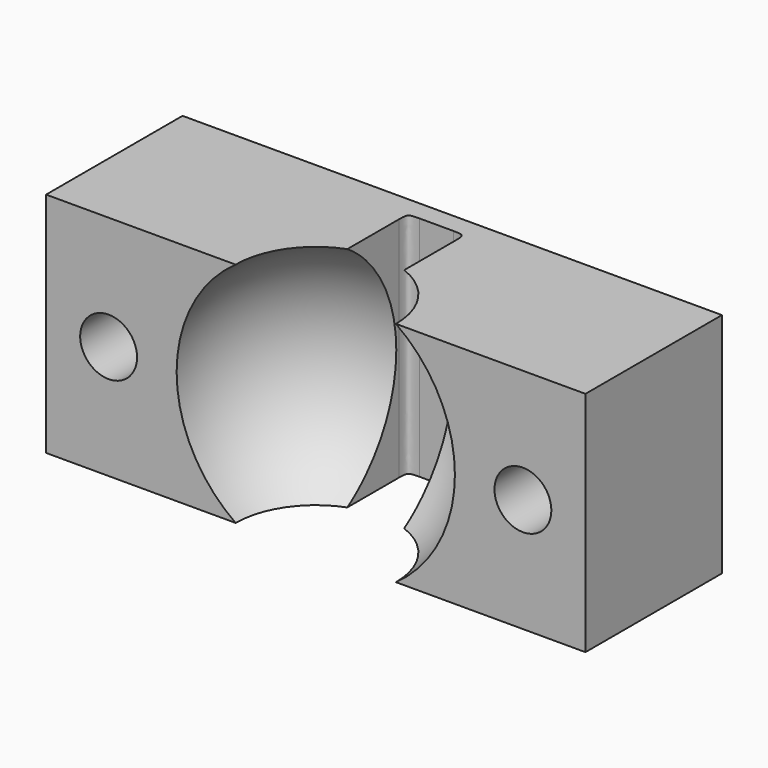
from build123d import *

# Parameters (mm, degrees)
F0_W        = 47.4317967892
F0_H        = 20
F0_R        = 4.5
F1_DEPTH    = 15
F2_R        = 7.05
F3_DEPTH    = 25
F7_DEPTH    = 13.25
F8_T1_DEPTH = 20
F9_START    = 10
F0_R_2      = 2.5
F9_DEPTH    = 5


# Not quite as in the source:
# - a fillet or chamfer that OpenCascade refuses, or shapes differently, is made with other operations: its cross-section is extruded or revolved along the edge and cut away or added


with BuildPart() as f1:
    # F0 (on Front) → F1 (new body)
    with BuildSketch(Plane.XZ):
        Rectangle(F0_W, F0_H)
        with Locations((-18.2158983946, 0)):
            Circle(F0_R, mode=Mode.SUBTRACT)
        with Locations((18.2158983946, 0)):
            Circle(F0_R, mode=Mode.SUBTRACT)
    extrude(amount=F1_DEPTH)

    # F2 (on face) → F3 (cut)
    with BuildSketch(Plane.XY.offset(10)):
        with Locations((0, -15)):
            Circle(F2_R)
    extrude(amount=-F3_DEPTH, mode=Mode.SUBTRACT)

    # F4 (on face) → F5 (revolve, cut)
    with BuildSketch(Plane.XZ.offset(15)):
        with BuildLine():
            Line((-7.05, -10), (-7.05, 10))
            ThreePointArc((-7.05, 10), (-12.2352972992, 0), (-7.05, -10))
        make_face()
    revolve(axis=Axis((0, -15, 0.0368109904), (0, 0, -1)), mode=Mode.SUBTRACT)

    # F6 (on face) → F7 (cut)
    with BuildSketch(Plane.XZ.offset(15)):
        Polygon((2.5, -10.0813228637), (2.5, 10), (0, 10), (-2.5, 10), (-2.5, -10.0813228637), (0, -10.0813228637), align=None)
    extrude(amount=-F7_DEPTH, mode=Mode.SUBTRACT)

    # F8: fillet of radius 1 on 2 edges, made by hand

    # F8_s2 → F8_t1 (join)
    with BuildSketch(Plane.XY.offset(-10)):
        with BuildLine():
            add(Edge.make_bspline(
                [(1.5, -1.75), (2.5, -1.75), (2.5, -2.75)],
                knots=[0, 0, 0, 1, 1, 1], degree=2, weights=[1, 2.3333333333, 1]))
            Line((2.5, -2.75), (2.5, -1.75))
            Line((2.5, -1.75), (1.5, -1.75))
        make_face()
        with BuildLine():
            add(Edge.make_bspline(
                [(-2.5, -2.75), (-2.5, -1.75), (-1.5, -1.75)],
                knots=[0, 0, 0, 1, 1, 1], degree=2, weights=[1, 2.3333333333, 1]))
            Line((-1.5, -1.75), (-2.5, -1.75))
            Line((-2.5, -1.75), (-2.5, -2.75))
        make_face()
    extrude(amount=F8_T1_DEPTH)

    # F0 (on Front) → F9 (join)
    with BuildSketch(Plane.XZ.offset(F9_START)):
        with Locations((-18.2158983946, 0)):
            Circle(F0_R)
        with Locations((-18.2158983946, 0)):
            Circle(F0_R_2, mode=Mode.SUBTRACT)
        with Locations((18.2158983946, 0)):
            Circle(F0_R)
        with Locations((18.2158983946, 0)):
            Circle(F0_R_2, mode=Mode.SUBTRACT)
    extrude(amount=F9_DEPTH)


solid = f1.part
